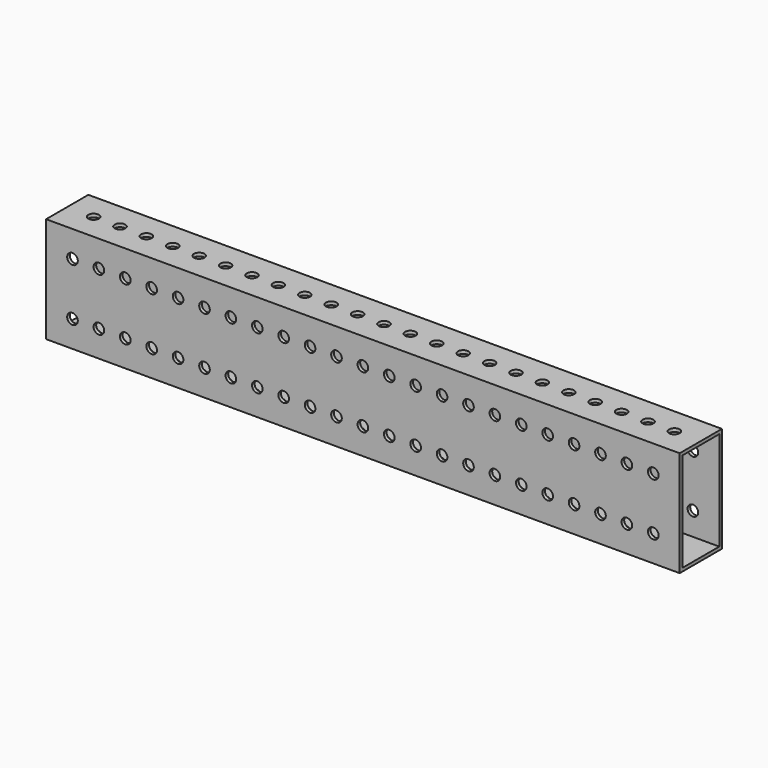
from build123d import *

# Parameters (mm, degrees)
F0_W     = 25.4
F0_H     = 50.8
F0_W_2   = 22.225
F0_H_2   = 47.625
F1_DEPTH = 304.8
F2_R     = 2.5527
F3_DEPTH = 254
F4_R     = 2.5527
F5_DEPTH = 76.2


# Not quite as in the source:
# - a feature names something its author has since deleted; it is built from what else it names


with BuildPart() as f1:
    # F0 (on Right) → F1 (new body)
    with BuildSketch(Plane.YZ):
        Rectangle(F0_W, F0_H)
        Rectangle(F0_W_2, F0_H_2, mode=Mode.SUBTRACT)
    extrude(amount=F1_DEPTH)

    # F2 (on face) → F3 (cut)
    with BuildSketch(Plane.XY.offset(25.4)):
        with Locations((12.7, 0)):
            Circle(F2_R)
        with Locations((25.4, 0)):
            Circle(F2_R)
        with Locations((38.1, 0)):
            Circle(F2_R)
        with Locations((50.8, 0)):
            Circle(F2_R)
        with Locations((63.5, 0)):
            Circle(F2_R)
        with Locations((76.2, 0)):
            Circle(F2_R)
        with Locations((88.9, 0)):
            Circle(F2_R)
        with Locations((101.6, 0)):
            Circle(F2_R)
        with Locations((114.3, 0)):
            Circle(F2_R)
        with Locations((127, 0)):
            Circle(F2_R)
        with Locations((139.7, 0)):
            Circle(F2_R)
        with Locations((152.4, 0)):
            Circle(F2_R)
        with Locations((165.1, 0)):
            Circle(F2_R)
        with Locations((177.8, 0)):
            Circle(F2_R)
        with Locations((190.5, 0)):
            Circle(F2_R)
        with Locations((203.2, 0)):
            Circle(F2_R)
        with Locations((215.9, 0)):
            Circle(F2_R)
        with Locations((228.6, 0)):
            Circle(F2_R)
        with Locations((241.3, 0)):
            Circle(F2_R)
        with Locations((254, 0)):
            Circle(F2_R)
        with Locations((266.7, 0)):
            Circle(F2_R)
        with Locations((279.4, 0)):
            Circle(F2_R)
        with Locations((292.1, 0)):
            Circle(F2_R)
    extrude(amount=-F3_DEPTH, mode=Mode.SUBTRACT)

    # F4 (on face) → F5 (cut)
    with BuildSketch(Plane.XZ.offset(12.7)):
        with Locations((114.3, 12.7)):
            Circle(F4_R)
        with Locations((177.8, 12.7)):
            Circle(F4_R)
        with Locations((25.4, -12.7)):
            Circle(F4_R)
        with Locations((12.7, 12.7)):
            Circle(F4_R)
        with Locations((241.3, -12.7)):
            Circle(F4_R)
        with Locations((254, -12.7)):
            Circle(F4_R)
        with Locations((139.7, 12.7)):
            Circle(F4_R)
        with Locations((38.1, -12.7)):
            Circle(F4_R)
        with Locations((215.9, 12.7)):
            Circle(F4_R)
        with Locations((76.2, 12.7)):
            Circle(F4_R)
        with Locations((241.3, 12.7)):
            Circle(F4_R)
        with Locations((292.1, 12.7)):
            Circle(F4_R)
        with Locations((127, 12.7)):
            Circle(F4_R)
        with Locations((101.6, -12.7)):
            Circle(F4_R)
        with Locations((279.4, 12.7)):
            Circle(F4_R)
        with Locations((165.1, -12.7)):
            Circle(F4_R)
        with Locations((165.1, 12.7)):
            Circle(F4_R)
        with Locations((152.4, -12.7)):
            Circle(F4_R)
        with Locations((266.7, 12.7)):
            Circle(F4_R)
        with Locations((63.5, -12.7)):
            Circle(F4_R)
        with Locations((215.9, -12.7)):
            Circle(F4_R)
        with Locations((177.8, -12.7)):
            Circle(F4_R)
        with Locations((254, 12.7)):
            Circle(F4_R)
        with Locations((228.6, 12.7)):
            Circle(F4_R)
        with Locations((152.4, 12.7)):
            Circle(F4_R)
        with Locations((38.1, 12.7)):
            Circle(F4_R)
        with Locations((12.7, -12.7)):
            Circle(F4_R)
        with Locations((139.7, -12.7)):
            Circle(F4_R)
        with Locations((266.7, -12.7)):
            Circle(F4_R)
        with Locations((279.4, -12.7)):
            Circle(F4_R)
        with Locations((127, -12.7)):
            Circle(F4_R)
        with Locations((25.4, 12.7)):
            Circle(F4_R)
        with Locations((190.5, -12.7)):
            Circle(F4_R)
        with Locations((50.8, 12.7)):
            Circle(F4_R)
        with Locations((101.6, 12.7)):
            Circle(F4_R)
        with Locations((228.6, -12.7)):
            Circle(F4_R)
        with Locations((50.8, -12.7)):
            Circle(F4_R)
        with Locations((88.9, 12.7)):
            Circle(F4_R)
        with Locations((190.5, 12.7)):
            Circle(F4_R)
        with Locations((114.3, -12.7)):
            Circle(F4_R)
        with Locations((88.9, -12.7)):
            Circle(F4_R)
        with Locations((203.2, -12.7)):
            Circle(F4_R)
        with Locations((76.2, -12.7)):
            Circle(F4_R)
        with Locations((63.5, 12.7)):
            Circle(F4_R)
        with Locations((203.2, 12.7)):
            Circle(F4_R)
        with Locations((292.1, -12.7)):
            Circle(F4_R)
    extrude(amount=-F5_DEPTH, mode=Mode.SUBTRACT)


solid = f1.part
